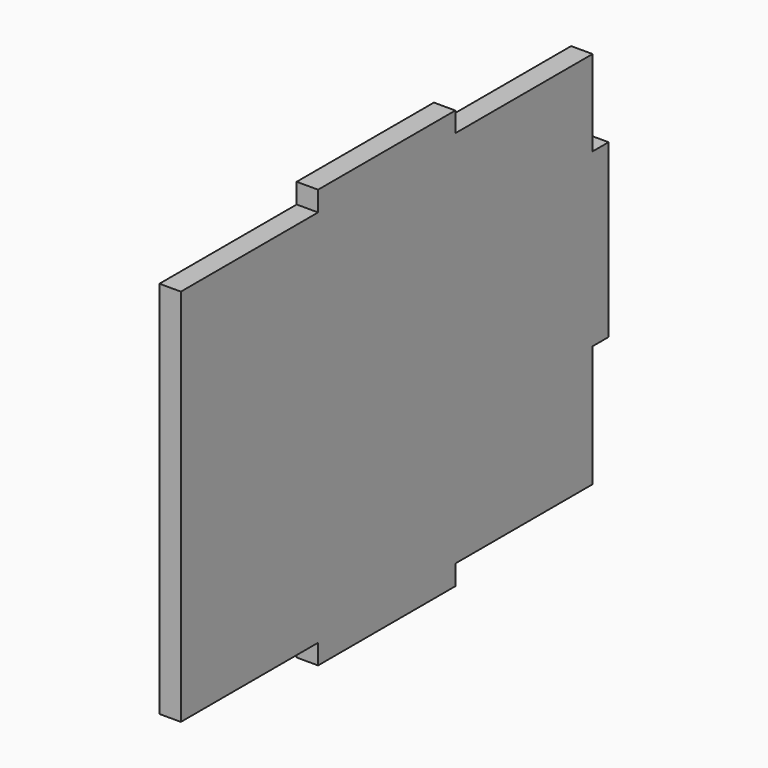
from build123d import *

# Parameters (mm, degrees)
F0_W     = 152.4
F0_H     = 17.78
F0_W_2   = 17.78
F0_H_2   = 152.4
F1_DEPTH = 19.05


# Not quite as in the source:
# - a feature names something its author has since deleted; it is built from what else it names


with BuildPart() as f1:
    # F0 (on Right) → F1 (new body)
    with BuildSketch(Plane.YZ):
        with Locations((0, 8.89)):
            Rectangle(F0_W, F0_H)
        Polygon((-76.2, 0), (-228.6, 0), (-228.6, -336.55), (-76.2, -336.55), (76.2, -336.55), (228.6, -336.55), (228.6, -228.6), (228.6, -76.2), (228.6, 0), (76.2, 0), align=None)
        with Locations((237.49, -152.4)):
            Rectangle(F0_W_2, F0_H_2)
        with Locations((0, -345.44)):
            Rectangle(F0_W, F0_H)
    extrude(amount=F1_DEPTH)


solid = f1.part
